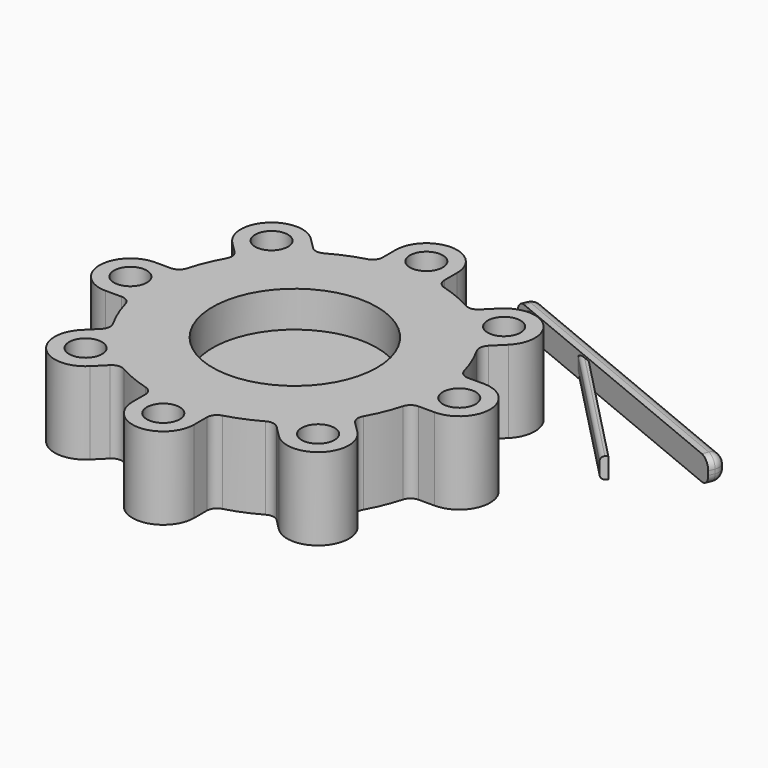
from build123d import *

# Parameters (mm, degrees)
F0_R      = 40
F0_R_2    = 8
F1_DEPTH  = 20
F3_DEPTH  = 5
F4_R      = 4.999
F5_W      = 150
F5_H      = 12
F6_DEPTH  = 8
F7_R      = 5
F9_DEPTH  = 5
F10_R     = 2
F11_R     = 40
F12_DEPTH = 2.5


# Not quite as in the source:
# - a fillet or chamfer is up to 0.001 mm smaller than in the source, because OpenCascade refuses the exact size


with BuildPart() as f1:
    # F0 (on Top) → F1 (new body, symmetric)
    with BuildSketch(Plane.XY):
        with BuildLine():
            ThreePointArc((-15, 72.284161474), (-16.0208878712, 69.2565111199), (-18.6666666667, 67.4652173757))
            ThreePointArc((-18.6666666667, 67.4652173757), (-26.7878402656, 64.6715672758), (-34.5057861185, 60.9044392828))
            ThreePointArc((-34.5057861185, 60.9044392828), (-49.4974746831, 49.4974746831), (-60.9044392828, 34.5057861185))
            ThreePointArc((-60.9044392828, 34.5057861185), (-64.6715672758, 26.7878402656), (-67.4652173757, 18.6666666667))
            ThreePointArc((-67.4652173757, 18.6666666667), (-70, 0), (-67.4652173757, -18.6666666667))
            ThreePointArc((-67.4652173757, -18.6666666667), (-64.6715672758, -26.7878402656), (-60.9044392828, -34.5057861185))
            ThreePointArc((-60.9044392828, -34.5057861185), (-49.4974746831, -49.4974746831), (-34.5057861185, -60.9044392828))
            ThreePointArc((-34.5057861185, -60.9044392828), (-26.7878402656, -64.6715672758), (-18.6666666667, -67.4652173757))
            ThreePointArc((-18.6666666667, -67.4652173757), (0, -70), (18.6666666667, -67.4652173757))
            ThreePointArc((18.6666666667, -67.4652173757), (26.7878402656, -64.6715672758), (34.5057861185, -60.9044392828))
            ThreePointArc((34.5057861185, -60.9044392828), (49.4974746831, -49.4974746831), (60.9044392828, -34.5057861185))
            ThreePointArc((60.9044392828, -34.5057861185), (64.6715672758, -26.7878402656), (67.4652173757, -18.6666666667))
            ThreePointArc((67.4652173757, -18.6666666667), (70, 0), (67.4652173757, 18.6666666667))
            ThreePointArc((67.4652173757, 18.6666666667), (64.6715672758, 26.7878402656), (60.9044392828, 34.5057861185))
            ThreePointArc((60.9044392828, 34.5057861185), (49.4974746831, 49.4974746831), (34.5057861185, 60.9044392828))
            ThreePointArc((34.5057861185, 60.9044392828), (26.7878402656, 64.6715672758), (18.6666666667, 67.4652173757))
            ThreePointArc((18.6666666667, 67.4652173757), (16.0208878712, 69.2565111199), (15, 72.284161474))
            Line((15, 72.284161474), (15, 80))
            ThreePointArc((15, 80), (0, 95), (-15, 80))
            Line((-15, 80), (-15, 72.284161474))
        make_face()
        Circle(F0_R, mode=Mode.SUBTRACT)
        with Locations((0, 80)):
            Circle(F0_R_2, mode=Mode.SUBTRACT)
        with BuildLine():
            ThreePointArc((-60.9044392828, 34.5057861185), (-49.4974746831, 49.4974746831), (-34.5057861185, 60.9044392828))
            ThreePointArc((-34.5057861185, 60.9044392828), (-37.6432701998, 60.3002271086), (-40.5060190329, 61.7192224685))
            Line((-40.5060190329, 61.7192224685), (-45.9619407771, 67.1751442127))
            ThreePointArc((-45.9619407771, 67.1751442127), (-67.1751442127, 67.1751442127), (-67.1751442127, 45.9619407771))
            Line((-67.1751442127, 45.9619407771), (-61.7192224685, 40.5060190329))
            ThreePointArc((-61.7192224685, 40.5060190329), (-60.3002271086, 37.6432701998), (-60.9044392828, 34.5057861185))
        make_face()
        with Locations((-56.5685424949, 56.5685424949)):
            Circle(F0_R_2, mode=Mode.SUBTRACT)
        with BuildLine():
            ThreePointArc((-67.4652173757, -18.6666666667), (-70, 0), (-67.4652173757, 18.6666666667))
            ThreePointArc((-67.4652173757, 18.6666666667), (-69.2565111199, 16.0208878712), (-72.284161474, 15))
            Line((-72.284161474, 15), (-80, 15))
            ThreePointArc((-80, 15), (-95, 0), (-80, -15))
            Line((-80, -15), (-72.284161474, -15))
            ThreePointArc((-72.284161474, -15), (-69.2565111199, -16.0208878712), (-67.4652173757, -18.6666666667))
        make_face()
        with Locations((-80, 0)):
            Circle(F0_R_2, mode=Mode.SUBTRACT)
        with BuildLine():
            ThreePointArc((-34.5057861185, -60.9044392828), (-49.4974746831, -49.4974746831), (-60.9044392828, -34.5057861185))
            ThreePointArc((-60.9044392828, -34.5057861185), (-60.3002271086, -37.6432701998), (-61.7192224685, -40.5060190329))
            Line((-61.7192224685, -40.5060190329), (-67.1751442127, -45.9619407771))
            ThreePointArc((-67.1751442127, -45.9619407771), (-67.1751442127, -67.1751442127), (-45.9619407771, -67.1751442127))
            Line((-45.9619407771, -67.1751442127), (-40.5060190329, -61.7192224685))
            ThreePointArc((-40.5060190329, -61.7192224685), (-37.6432701998, -60.3002271086), (-34.5057861185, -60.9044392828))
        make_face()
        with Locations((-56.5685424949, -56.5685424949)):
            Circle(F0_R_2, mode=Mode.SUBTRACT)
        with BuildLine():
            ThreePointArc((40.5060190329, 61.7192224685), (37.6432701998, 60.3002271086), (34.5057861185, 60.9044392828))
            ThreePointArc((34.5057861185, 60.9044392828), (49.4974746831, 49.4974746831), (60.9044392828, 34.5057861185))
            ThreePointArc((60.9044392828, 34.5057861185), (60.3002271086, 37.6432701998), (61.7192224685, 40.5060190329))
            Line((61.7192224685, 40.5060190329), (67.1751442127, 45.9619407771))
            ThreePointArc((67.1751442127, 45.9619407771), (67.1751442127, 67.1751442127), (45.9619407771, 67.1751442127))
            Line((45.9619407771, 67.1751442127), (40.5060190329, 61.7192224685))
        make_face()
        with Locations((56.5685424949, 56.5685424949)):
            Circle(F0_R_2, mode=Mode.SUBTRACT)
        with BuildLine():
            ThreePointArc((18.6666666667, -67.4652173757), (0, -70), (-18.6666666667, -67.4652173757))
            ThreePointArc((-18.6666666667, -67.4652173757), (-16.0208878712, -69.2565111199), (-15, -72.284161474))
            Line((-15, -72.284161474), (-15, -80))
            ThreePointArc((-15, -80), (0, -95), (15, -80))
            Line((15, -80), (15, -72.284161474))
            ThreePointArc((15, -72.284161474), (16.0208878712, -69.2565111199), (18.6666666667, -67.4652173757))
        make_face()
        with Locations((0, -80)):
            Circle(F0_R_2, mode=Mode.SUBTRACT)
        with BuildLine():
            ThreePointArc((72.284161474, 15), (69.2565111199, 16.0208878712), (67.4652173757, 18.6666666667))
            ThreePointArc((67.4652173757, 18.6666666667), (70, 0), (67.4652173757, -18.6666666667))
            ThreePointArc((67.4652173757, -18.6666666667), (69.2565111199, -16.0208878712), (72.284161474, -15))
            Line((72.284161474, -15), (80, -15))
            ThreePointArc((80, -15), (95, 0), (80, 15))
            Line((80, 15), (72.284161474, 15))
        make_face()
        with Locations((80, 0)):
            Circle(F0_R_2, mode=Mode.SUBTRACT)
        with BuildLine():
            ThreePointArc((60.9044392828, -34.5057861185), (49.4974746831, -49.4974746831), (34.5057861185, -60.9044392828))
            ThreePointArc((34.5057861185, -60.9044392828), (37.6432701998, -60.3002271086), (40.5060190329, -61.7192224685))
            Line((40.5060190329, -61.7192224685), (45.9619407771, -67.1751442127))
            ThreePointArc((45.9619407771, -67.1751442127), (67.1751442127, -67.1751442127), (67.1751442127, -45.9619407771))
            Line((67.1751442127, -45.9619407771), (61.7192224685, -40.5060190329))
            ThreePointArc((61.7192224685, -40.5060190329), (60.3002271086, -37.6432701998), (60.9044392828, -34.5057861185))
        make_face()
        with Locations((56.5685424949, -56.5685424949)):
            Circle(F0_R_2, mode=Mode.SUBTRACT)
    extrude(amount=F1_DEPTH, both=True)

    # F2 (on Top) → F3 (join, symmetric)
    with BuildSketch(Plane.XY):
        Polygon((43.7283586707, 92.5039669143), (34.4895633456, 96.330801238), (16.6130997625, 53.1732004085), (25.8518950877, 49.3463660849), align=None)
    extrude(amount=F3_DEPTH, both=True)

    # F4 (radius 5 in the source; OpenCascade refuses exactly that, so slightly less here)
    f4_edges = [f1.edges().sort_by_distance(p)[0] for p in [
        (37.533586, 77.548464, 5),
        (28.294791, 81.375298, 5),
        (28.294791, 81.375298, -5),
        (37.533586, 77.548464, -5),
    ]]
    fillet(f4_edges, radius=F4_R)

    # F5 (on face) → F6 (join)
    with BuildSketch(Plane(origin=(39.1089610081, 94.4173840762, 0), x_dir=(-0.9238795325, 0.3826834324, 0), z_dir=(0.3826834324, 0.9238795325, 0))):
        with Locations((-65, 0)):
            Rectangle(F5_W, F5_H)
        with BuildLine():
            Line((-5, -0.001), (-5, 0.001))
            ThreePointArc((-5, 0.001), (-3.5358267992, 3.5358267992), (-0.001, 5))
            Line((-0.001, 5), (0.001, 5))
            ThreePointArc((0.001, 5), (3.5358267992, 3.5358267992), (5, 0.001))
            Line((5, 0.001), (5, -0.001))
            ThreePointArc((5, -0.001), (3.5358267992, -3.5358267992), (0.001, -5))
            Line((0.001, -5), (-0.001, -5))
            ThreePointArc((-0.001, -5), (-3.5358267992, -3.5358267992), (-5, -0.001))
        make_face(mode=Mode.SUBTRACT)
        with BuildLine():
            ThreePointArc((-0.001, 5), (-3.5358267992, 3.5358267992), (-5, 0.001))
            Line((-5, 0.001), (-5, -0.001))
            ThreePointArc((-5, -0.001), (-3.5358267992, -3.5358267992), (-0.001, -5))
            Line((-0.001, -5), (0.001, -5))
            ThreePointArc((0.001, -5), (3.5358267992, -3.5358267992), (5, -0.001))
            Line((5, -0.001), (5, 0.001))
            ThreePointArc((5, 0.001), (3.5358267992, 3.5358267992), (0.001, 5))
            Line((0.001, 5), (-0.001, 5))
        make_face()
    extrude(amount=F6_DEPTH)

    # F7
    f7_edges = [f1.edges().sort_by_distance(p)[0] for p in [
        (31.400899, 101.939737, 6),
        (31.400899, 101.939737, -6),
        (102.222598, 76.933997, 6),
        (102.222598, 76.933997, -6),
        (32.931633, 105.635255, 0),
        (171.513563, 48.23274, 0),
        (169.982829, 44.537222, 6),
        (169.982829, 44.537222, -6),
    ]]
    fillet(f7_edges, radius=F7_R)

    # F8 (on Top) → F9 (join, symmetric)
    with BuildSketch(Plane.XY):
        Polygon((81.5432720327, 76.8405169398), (73.8736570753, 80.0173754734), (133.6454618744, 18.3365114568), (136.0131502151, 20.6309184432), align=None)
    extrude(amount=F9_DEPTH, both=True)

    # F10
    f10_edges = [f1.edges().sort_by_distance(p)[0] for p in [
        (103.759559, 49.176943, 5),
        (103.759559, 49.176943, -5),
    ]]
    fillet(f10_edges, radius=F10_R)

    # F11 (on Top) → F12 (join, symmetric)
    with BuildSketch(Plane.XY):
        Circle(F11_R)
    extrude(amount=F12_DEPTH, both=True)


solid = f1.part
